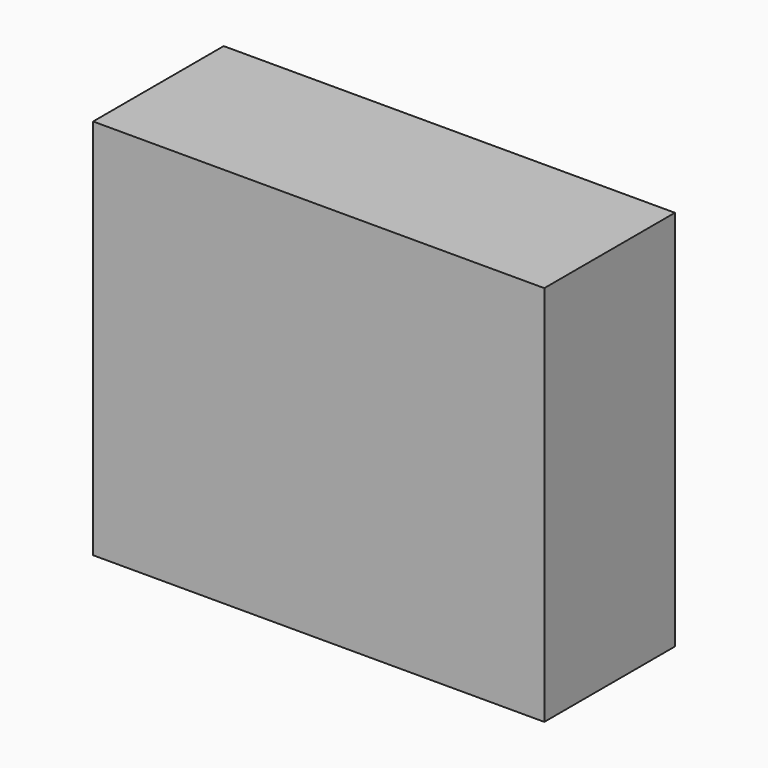
from build123d import *

# Parameters (mm, degrees)
F0_W     = 70.2064186335
F0_H     = 59.4210922718
F2_DEPTH = 25.4
F3_DEPTH = 12.9629038274


# Not quite as in the source:
# - the program builds the solid bodies; features that only make, move or delete a surface that nothing else refers to are left out


with BuildPart() as f2:
    # F0 (on Front) → F2 (new body)
    with BuildSketch(Plane.XZ):
        with Locations((35.1032093167, 29.7105461359)):
            Rectangle(F0_W, F0_H)
    extrude(amount=F2_DEPTH)

    # F1 (on face) → F3 (join)
    with BuildSketch(Plane.XZ):
        with BuildLine():
            Line((25.4531949759, 29.8861153424), (40.9622192383, 44.9872016907))
            ThreePointArc((40.9622192383, 44.9872016907), (18.2216341505, 52.8275624371), (25.4531949759, 29.8861153424))
        make_face()
    extrude(amount=F3_DEPTH)


solid = f2.part
